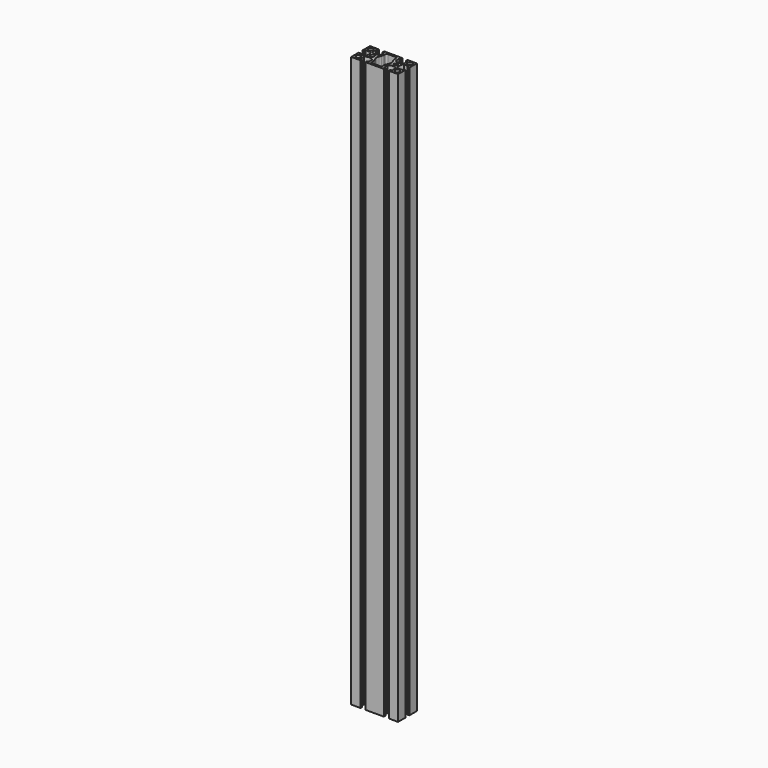
from build123d import *

# Parameters (mm, degrees)
F0_R     = 3
F0_R_2   = 2.5
F1_DEPTH = 730.5
F2_R     = 2
F3_R     = 7


# Not quite as in the source:
# - a feature names something its author has since deleted; it is built from what else it names


with BuildPart() as f1:
    # F0 (on Top) → F1 (new body)
    with BuildSketch(Plane.XY):
        with BuildLine():
            Line((18.15, -15), (30, -15))
            Line((30, -15), (30, -3.15))
            Line((30, -3.15), (27.5, -3.15))
            Line((27.5, -3.15), (27.5, -5.15))
            Line((27.5, -5.15), (21.5477069044, -5.15))
            ThreePointArc((21.5477069044, -5.15), (19.5, 0), (21.5477069044, 5.15))
            Line((21.5477069044, 5.15), (27.5, 5.15))
            Line((27.5, 5.15), (27.5, 3.15))
            Line((27.5, 3.15), (30, 3.15))
            Line((30, 3.15), (30, 15))
            Line((30, 15), (18.15, 15))
            Line((18.15, 15), (18.15, 12.5))
            Line((18.15, 12.5), (20.15, 12.5))
            Line((20.15, 12.5), (20.15, 6.5477069044))
            ThreePointArc((20.15, 6.5477069044), (15, 4.5), (9.85, 6.5477069044))
            Line((9.85, 6.5477069044), (9.85, 12.5))
            Line((9.85, 12.5), (11.85, 12.5))
            Line((11.85, 12.5), (11.85, 15))
            Line((11.85, 15), (-11.85, 15))
            Line((-11.85, 15), (-11.85, 12.5))
            Line((-11.85, 12.5), (-9.85, 12.5))
            Line((-9.85, 12.5), (-9.85, 6.5477069044))
            ThreePointArc((-9.85, 6.5477069044), (-15, 4.5), (-20.15, 6.5477069044))
            Line((-20.15, 6.5477069044), (-20.15, 12.5))
            Line((-20.15, 12.5), (-18.15, 12.5))
            Line((-18.15, 12.5), (-18.15, 15))
            Line((-18.15, 15), (-30, 15))
            Line((-30, 15), (-30, 3.15))
            Line((-30, 3.15), (-27.5, 3.15))
            Line((-27.5, 3.15), (-27.5, 5.15))
            Line((-27.5, 5.15), (-21.5477069044, 5.15))
            ThreePointArc((-21.5477069044, 5.15), (-19.5, 0), (-21.5477069044, -5.15))
            Line((-21.5477069044, -5.15), (-27.5, -5.15))
            Line((-27.5, -5.15), (-27.5, -3.15))
            Line((-27.5, -3.15), (-30, -3.15))
            Line((-30, -3.15), (-30, -15))
            Line((-30, -15), (-18.15, -15))
            Line((-18.15, -15), (-18.15, -12.5))
            Line((-18.15, -12.5), (-20.15, -12.5))
            Line((-20.15, -12.5), (-20.15, -6.5477069044))
            ThreePointArc((-20.15, -6.5477069044), (-15, -4.5), (-9.85, -6.5477069044))
            Line((-9.85, -6.5477069044), (-9.85, -12.5))
            Line((-9.85, -12.5), (-11.85, -12.5))
            Line((-11.85, -12.5), (-11.85, -15))
            Line((-11.85, -15), (11.85, -15))
            Line((11.85, -15), (11.85, -12.5))
            Line((11.85, -12.5), (9.85, -12.5))
            Line((9.85, -12.5), (9.85, -6.5477069044))
            ThreePointArc((9.85, -6.5477069044), (15, -4.5), (20.15, -6.5477069044))
            Line((20.15, -6.5477069044), (20.15, -12.5))
            Line((20.15, -12.5), (18.15, -12.5))
            Line((18.15, -12.5), (18.15, -15))
        make_face()
        with Locations((-25, -10)):
            Circle(F0_R, mode=Mode.SUBTRACT)
        with Locations((25, -10)):
            Circle(F0_R, mode=Mode.SUBTRACT)
        with Locations((-15, 0)):
            Circle(F0_R_2, mode=Mode.SUBTRACT)
        with Locations((-25, 10)):
            Circle(F0_R, mode=Mode.SUBTRACT)
        Polygon((-7, 7), (-7, 12.5), (0, 12.5), (7, 12.5), (7, 7), (10, 0), (7, -7), (7, -12.5), (0, -12.5), (-7, -12.5), (-7, -7), (-10, 0), align=None, mode=Mode.SUBTRACT)
        with Locations((15, 0)):
            Circle(F0_R_2, mode=Mode.SUBTRACT)
        with Locations((25, 10)):
            Circle(F0_R, mode=Mode.SUBTRACT)
    extrude(amount=F1_DEPTH)

    # F2
    f2_edges = [f1.edges().sort_by_distance(p)[0] for p in [
        (-7, 12.5, 365.25),
        (7, 12.5, 365.25),
    ]]
    fillet(f2_edges, radius=F2_R)

    # F3
    f3_edges = [f1.edges().sort_by_distance(p)[0] for p in [
        (-7, 7, 365.25),
        (-10, 0, 365.25),
        (7, 7, 365.25),
        (10, 0, 365.25),
    ]]
    fillet(f3_edges, radius=F3_R)


solid = f1.part
